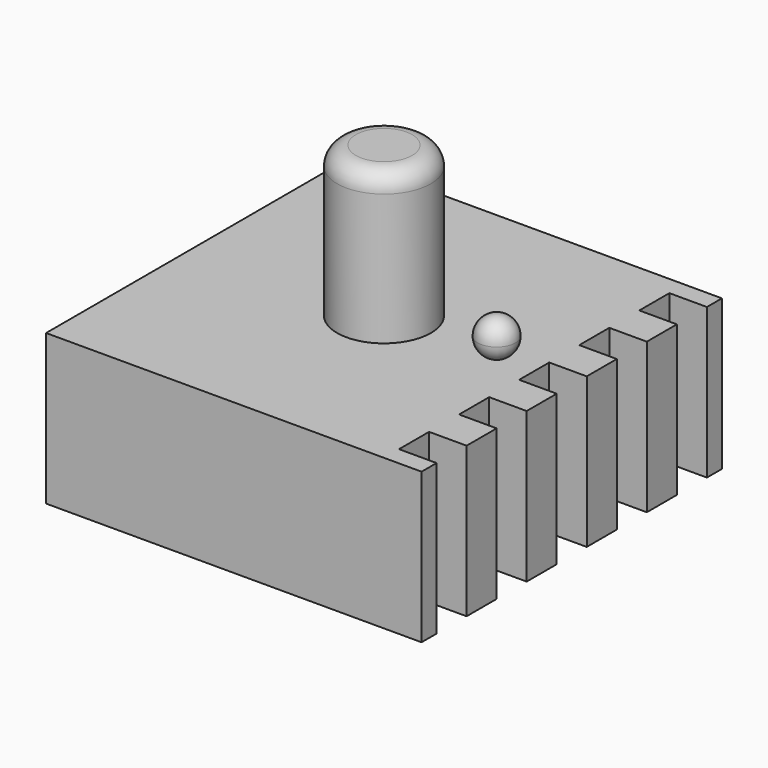
from build123d import *

# Parameters (mm, degrees)
F0_W      = 100
F0_H      = 100
F1_DEPTH  = 40
F3_R      = 12.5
F4_DEPTH  = 20
F5_DEPTH  = 40
F6_R      = 5
F7_W      = 10
F7_H      = 10
F8_DEPTH  = 40
F9_R      = 5
F10_DEPTH = 10
F11_R     = 4.99999


# Not quite as in the source:
# - a fillet or chamfer is up to 0.001 mm smaller than in the source, because OpenCascade refuses the exact size
# - a feature names something its author has since deleted; it is built from what else it names


with BuildPart() as f1:
    # F0 (on Top) → F1 (new body)
    with BuildSketch(Plane.XY):
        Rectangle(F0_W, F0_H)
    extrude(amount=F1_DEPTH)

    # F3 (on offset) → F4 (cut)
    with BuildSketch(Plane.XY.offset(40)):
        Circle(F3_R)
    extrude(amount=-F4_DEPTH, mode=Mode.SUBTRACT)

    # F7 (on face) → F8 (cut)
    with BuildSketch(Plane.XY.offset(40)):
        with Locations((45, 40)):
            Rectangle(F7_W, F7_H)
        with Locations((45, 20)):
            Rectangle(F7_W, F7_H)
        with Locations((45, 0)):
            Rectangle(F7_W, F7_H)
        with Locations((45, -20)):
            Rectangle(F7_W, F7_H)
        with Locations((45, -40)):
            Rectangle(F7_W, F7_H)
    extrude(amount=-F8_DEPTH, mode=Mode.SUBTRACT)


with BuildPart() as f5:
    # F3 (on offset) → F5 (new body)
    with BuildSketch(Plane.XY.offset(40)):
        Circle(F3_R)
    extrude(amount=F5_DEPTH)

    # F6
    f6_edges = [f5.edges().sort_by_distance(p)[0] for p in [
        (-12.5, 0, 80),
    ]]
    fillet(f6_edges, radius=F6_R)


with BuildPart() as f10:
    # F9 (on offset) → F10 (new body)
    with BuildSketch(Plane.XY.offset(40)):
        with Locations((30, 0)):
            Circle(F9_R)
    extrude(amount=F10_DEPTH)

    # F11 (radius 5 in the source; OpenCascade refuses exactly that, so slightly less here)
    f11_edges = [f10.edges().sort_by_distance(p)[0] for p in [
        (25, 0, 50),
        (35, 0, 45),
        (25, 0, 40),
    ]]
    fillet(f11_edges, radius=F11_R)


solid = Compound([f1.part, f5.part, f10.part])
